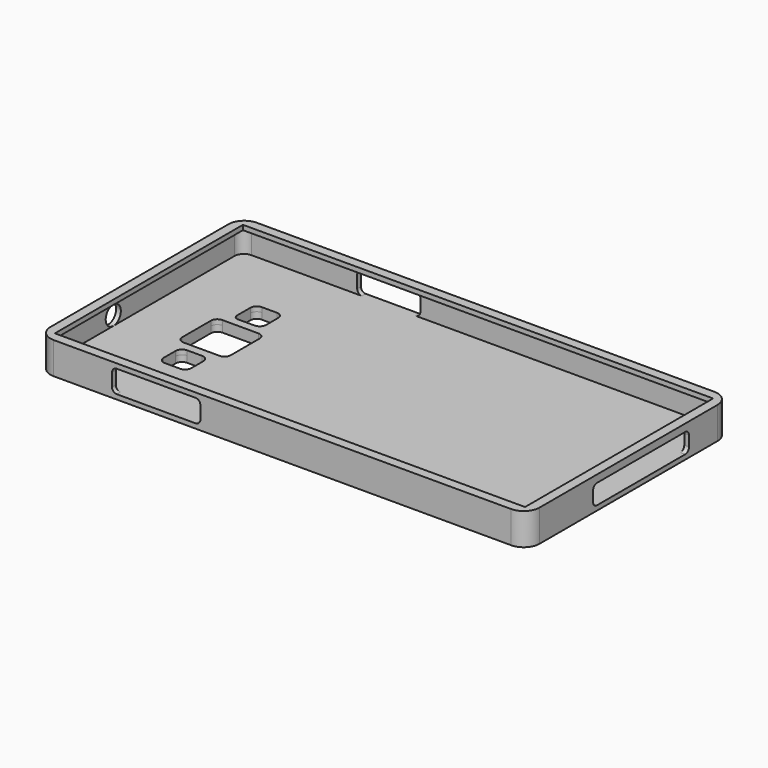
from build123d import *

# Parameters (mm, degrees)
F0_W      = 155
F0_H      = 80.5
F1_DEPTH  = 8.6
F2_T      = -1.5
F3_W      = 155
F3_H      = 80.5
F3_W_2    = 152
F3_H_2    = 77.5
F3_W_3    = 149
F3_H_3    = 74.5
F4_DEPTH  = 1.5
F5_W      = 28
F5_H      = 7.1
F6_DEPTH  = 1.5
F7_W      = 20
F7_H      = 7.1
F8_DEPTH  = 1.5
F9_R      = 3
F10_DEPTH = 1.5
F11_W     = 38
F11_H     = 6.2492947091
F12_DEPTH = 1.5
F13_W     = 8.8
F13_H     = 4.4
F13_W_2   = 15.4
F13_H_2   = 7.7
F14_DEPTH = 1.5
F15_R     = 1.5
F16_R     = 2
F17_R     = 5
F18_R     = 3
F20_DEPTH = 2
F21_R     = 1.99999
F23_DEPTH = 2
F24_R     = 1.5
F25_DEPTH = 2
F26_R     = 1.5


# Not quite as in the source:
# - a fillet or chamfer is up to 0.001 mm smaller than in the source, because OpenCascade refuses the exact size


with BuildPart() as f1:
    # F0 (on Top) → F1 (new body)
    with BuildSketch(Plane.XY):
        with Locations((77.5, 40.25)):
            Rectangle(F0_W, F0_H)
    extrude(amount=F1_DEPTH)

    # F2
    f2_openings = [f1.faces().sort_by_distance(p)[0] for p in [
        (77.5, 40.25, 8.6),
    ]]
    offset(amount=F2_T, openings=f2_openings)

    # F3 (on face) → F4 (join)
    with BuildSketch(Plane.XY.offset(8.6)):
        with Locations((77.5, 40.25)):
            Rectangle(F3_W, F3_H)
        with Locations((77.5, 40.25)):
            Rectangle(F3_W_2, F3_H_2, mode=Mode.SUBTRACT)
        with Locations((77.5, 40.25)):
            Rectangle(F3_W_2, F3_H_2)
        with Locations((77.5, 40.25)):
            Rectangle(F3_W_3, F3_H_3, mode=Mode.SUBTRACT)
    extrude(amount=F4_DEPTH)

    # F5 (on face) → F6 (cut, through all)
    with BuildSketch(Plane.XZ):
        with Locations((37.5, 5.05)):
            Rectangle(F5_W, F5_H)
    extrude(amount=-F6_DEPTH, mode=Mode.SUBTRACT)

    # F7 (on face) → F8 (cut, through all)
    with BuildSketch(Plane(origin=(0, 80.5, 0), x_dir=(-1, 0, 0), z_dir=(0, 1, 0))):
        with Locations((-48, 5.05)):
            Rectangle(F7_W, F7_H)
    extrude(amount=-F8_DEPTH, mode=Mode.SUBTRACT)

    # F9 (on face) → F10 (cut, through all)
    with BuildSketch(Plane(origin=(0, 0, 0), x_dir=(0, -1, 0), z_dir=(-1, 0, 0))):
        with Locations((-28, 4.5)):
            Circle(F9_R)
    extrude(amount=-F10_DEPTH, mode=Mode.SUBTRACT)

    # F11 (on face) → F12 (cut, through all)
    with BuildSketch(Plane.YZ.offset(155)):
        with Locations((45.2, 4.6246473546)):
            Rectangle(F11_W, F11_H)
    extrude(amount=-F12_DEPTH, mode=Mode.SUBTRACT)

    # F13 (on face) → F14 (cut, through all)
    with BuildSketch(Plane(origin=(0, 0, 0), x_dir=(1, 0, 0), z_dir=(0, 0, -1))):
        with Locations((26.2872223049, -27.05)):
            Rectangle(F13_W, F13_H)
        with Locations((26.2872223049, -22.65)):
            Rectangle(F13_W, F13_H)
        with Locations((26.2872223049, -35.8)):
            Rectangle(F13_W_2, F13_H_2)
        with Locations((26.2872223049, -43.5)):
            Rectangle(F13_W_2, F13_H_2)
        with Locations((26.2872223049, -52.25)):
            Rectangle(F13_W, F13_H)
        with Locations((26.2872223049, -56.65)):
            Rectangle(F13_W, F13_H)
    extrude(amount=-F14_DEPTH, mode=Mode.SUBTRACT)

    # F15
    f15_edges = [f1.edges().sort_by_distance(p)[0] for p in [
        (23.5, 0.75, 8.6),
        (51.5, 0.75, 8.6),
        (51.5, 0.75, 1.5),
        (23.5, 0.75, 1.5),
        (154.25, 26.2, 7.749295),
        (154.25, 26.2, 1.5),
        (154.25, 64.2, 7.749295),
        (154.25, 64.2, 1.5),
        (58, 79.75, 8.6),
        (58, 79.75, 1.5),
        (38, 79.75, 8.6),
        (38, 79.75, 1.5),
        (21.887222, 50.05, 0.75),
    ]]
    fillet(f15_edges, radius=F15_R)

    # F16
    f16_edges = [f1.edges().sort_by_distance(p)[0] for p in [
        (21.887222, 29.25, 0.75),
        (18.587222, 47.35, 0.75),
        (21.887222, 58.85, 0.75),
        (21.887222, 20.45, 0.75),
        (18.587222, 31.95, 0.75),
        (30.687222, 50.05, 0.75),
        (33.987222, 31.95, 0.75),
        (30.687222, 20.45, 0.75),
        (30.687222, 29.25, 0.75),
        (33.987222, 47.35, 0.75),
        (30.687222, 58.85, 0.75),
    ]]
    fillet(f16_edges, radius=F16_R)

    # F17
    f17_edges = [f1.edges().sort_by_distance(p)[0] for p in [
        (0, 0, 5.05),
        (0, 80.5, 5.05),
        (155, 0, 5.05),
        (155, 80.5, 5.05),
    ]]
    fillet(f17_edges, radius=F17_R)

    # F18
    f18_edges = [f1.edges().sort_by_distance(p)[0] for p in [
        (1.5, 79, 5.05),
        (1.5, 1.5, 5.05),
        (153.5, 79, 5.05),
        (153.5, 1.5, 5.05),
    ]]
    fillet(f18_edges, radius=F18_R)

    # F19 (on face) → F20 (join)
    with BuildSketch(Plane(origin=(0, 0, 0), x_dir=(1, 0, 0), z_dir=(0, 0, -1))):
        with BuildLine():
            Line((26.2872223049, -17.0733576864), (12.2872223049, -17.0733576864))
            Line((12.2872223049, -17.0733576864), (12.2872223049, -65.0733576864))
            Line((12.2872223049, -65.0733576864), (26.2872223049, -65.0733576864))
            Line((26.2872223049, -65.0733576864), (26.2872223049, -58.85))
            Line((26.2872223049, -58.85), (23.8872223049, -58.85))
            ThreePointArc((23.8872223049, -58.85), (22.4730087426, -58.2642135624), (21.8872223049, -56.85))
            Line((21.8872223049, -56.85), (21.8872223049, -51.55))
            ThreePointArc((21.8872223049, -51.55), (22.3265621332, -50.4893398282), (23.3872223049, -50.05))
            Line((23.3872223049, -50.05), (26.2872223049, -50.05))
            Line((26.2872223049, -50.05), (26.2872223049, -47.35))
            Line((26.2872223049, -47.35), (20.5872223049, -47.35))
            ThreePointArc((20.5872223049, -47.35), (19.1730087426, -46.7642135624), (18.5872223049, -45.35))
            Line((18.5872223049, -45.35), (18.5872223049, -33.95))
            ThreePointArc((18.5872223049, -33.95), (19.1730087426, -32.5357864376), (20.5872223049, -31.95))
            Line((20.5872223049, -31.95), (26.2872223049, -31.95))
            Line((26.2872223049, -31.95), (26.2872223049, -29.25))
            Line((26.2872223049, -29.25), (23.8872223049, -29.25))
            ThreePointArc((23.8872223049, -29.25), (22.4730087426, -28.6642135624), (21.8872223049, -27.25))
            Line((21.8872223049, -27.25), (21.8872223049, -22.45))
            ThreePointArc((21.8872223049, -22.45), (22.4730087426, -21.0357864376), (23.8872223049, -20.45))
            Line((23.8872223049, -20.45), (26.2872223049, -20.45))
            Line((26.2872223049, -20.45), (26.2872223049, -17.0733576864))
        make_face()
        with BuildLine():
            Line((40.2872223049, -17.0733576864), (26.2872223049, -17.0733576864))
            Line((26.2872223049, -17.0733576864), (26.2872223049, -20.45))
            Line((26.2872223049, -20.45), (28.6872223049, -20.45))
            ThreePointArc((28.6872223049, -20.45), (30.1014358673, -21.0357864376), (30.6872223049, -22.45))
            Line((30.6872223049, -22.45), (30.6872223049, -27.25))
            ThreePointArc((30.6872223049, -27.25), (30.1014358673, -28.6642135624), (28.6872223049, -29.25))
            Line((28.6872223049, -29.25), (26.2872223049, -29.25))
            Line((26.2872223049, -29.25), (26.2872223049, -31.95))
            Line((26.2872223049, -31.95), (31.9872223049, -31.95))
            ThreePointArc((31.9872223049, -31.95), (33.4014358673, -32.5357864376), (33.9872223049, -33.95))
            Line((33.9872223049, -33.95), (33.9872223049, -45.35))
            ThreePointArc((33.9872223049, -45.35), (33.4014358673, -46.7642135624), (31.9872223049, -47.35))
            Line((31.9872223049, -47.35), (26.2872223049, -47.35))
            Line((26.2872223049, -47.35), (26.2872223049, -50.05))
            Line((26.2872223049, -50.05), (28.6872223049, -50.05))
            ThreePointArc((28.6872223049, -50.05), (30.1014358673, -50.6357864376), (30.6872223049, -52.05))
            Line((30.6872223049, -52.05), (30.6872223049, -56.85))
            ThreePointArc((30.6872223049, -56.85), (30.1014358673, -58.2642135624), (28.6872223049, -58.85))
            Line((28.6872223049, -58.85), (26.2872223049, -58.85))
            Line((26.2872223049, -58.85), (26.2872223049, -65.0733576864))
            Line((26.2872223049, -65.0733576864), (40.2872223049, -65.0733576864))
            Line((40.2872223049, -65.0733576864), (40.2872223049, -17.0733576864))
        make_face()
    extrude(amount=F20_DEPTH)

    # F21 (radius 2 in the source; OpenCascade refuses exactly that, so slightly less here)
    f21_edges = [f1.edges().sort_by_distance(p)[0] for p in [
        (12.287222, 17.073358, -1),
        (40.287222, 17.073358, -1),
        (12.287222, 65.073358, -1),
        (40.287222, 65.073358, -1),
        (12.287222, 41.073358, -2),
        (26.287222, 65.073358, -2),
        (40.287222, 41.073358, -2),
        (26.287222, 17.073358, -2),
    ]]
    fillet(f21_edges, radius=F21_R)

    # F22 (on face) → F23 (join)
    with BuildSketch(Plane(origin=(0, 0, 0), x_dir=(1, 0, 0), z_dir=(0, 0, -1))):
        with BuildLine():
            ThreePointArc((139.0328407288, -9.85), (137.2650737758, -10.582233047), (136.5328407288, -12.35))
            Line((136.5328407288, -12.35), (136.5328407288, -40.25))
            Line((136.5328407288, -40.25), (141.5328407288, -40.25))
            Line((141.5328407288, -40.25), (141.5328407288, -12.35))
            ThreePointArc((141.5328407288, -12.35), (140.8006076817, -10.582233047), (139.0328407288, -9.85))
        make_face()
        with BuildLine():
            Line((141.5328407288, -40.25), (136.5328407288, -40.25))
            Line((136.5328407288, -40.25), (136.5328407288, -68.15))
            ThreePointArc((136.5328407288, -68.15), (137.2650737758, -69.917766953), (139.0328407288, -70.65))
            ThreePointArc((139.0328407288, -70.65), (140.8006076817, -69.917766953), (141.5328407288, -68.15))
            Line((141.5328407288, -68.15), (141.5328407288, -40.25))
        make_face()
    extrude(amount=F23_DEPTH)

    # F24
    f24_edges = [f1.edges().sort_by_distance(p)[0] for p in [
        (139.032841, 9.85, -2),
    ]]
    fillet(f24_edges, radius=F24_R)

    # F22 (on face) → F25 (join)
    with BuildSketch(Plane(origin=(0, 0, 0), x_dir=(1, 0, 0), z_dir=(0, 0, -1))):
        with BuildLine():
            ThreePointArc((81.033386401, -10.1015902981), (79.265619448, -10.8338233452), (78.533386401, -12.6015902981))
            Line((78.533386401, -12.6015902981), (78.533386401, -68.4015902981))
            ThreePointArc((78.533386401, -68.4015902981), (79.265619448, -70.1693572511), (81.033386401, -70.9015902981))
            ThreePointArc((81.033386401, -70.9015902981), (82.8011533539, -70.1693572511), (83.533386401, -68.4015902981))
            Line((83.533386401, -68.4015902981), (83.533386401, -12.6015902981))
            ThreePointArc((83.533386401, -12.6015902981), (82.8011533539, -10.8338233452), (81.033386401, -10.1015902981))
        make_face()
    extrude(amount=F25_DEPTH)

    # F26
    f26_edges = [f1.edges().sort_by_distance(p)[0] for p in [
        (78.533386, 40.50159, -2),
    ]]
    fillet(f26_edges, radius=F26_R)


solid = f1.part
